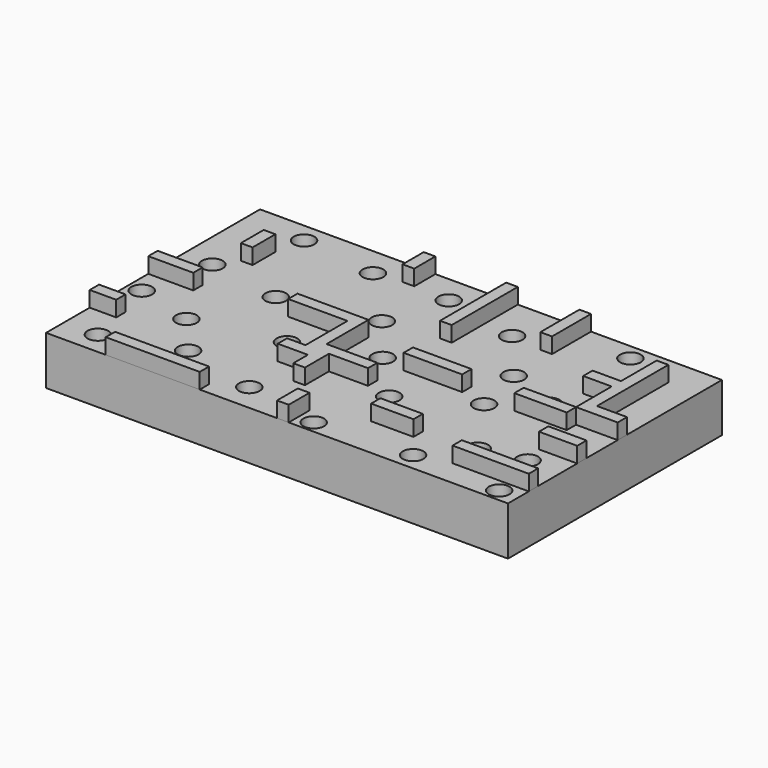
from build123d import *

# Parameters (mm, degrees)
F1_DEPTH = 12.7
F2_R     = 2.7051
F3_DEPTH = 12.701
F4_DEPTH = 12.701
F5_W     = 7.4367895722
F5_H     = 3.048
F6_DEPTH = 4.064
F5_W_2   = 13.6774629354
F5_W_3   = 9.984705162
F5_W_4   = 19.9265140414
F5_W_5   = 11.0705606639
F5_W_6   = 3.048
F5_H_2   = 6.795296824
F5_W_7   = 15.4987806454
F5_H_3   = 7.4474671856
F5_H_4   = 6.8967710249
F5_H_5   = 21.5904228389
F5_H_6   = 12.7339735627
F5_W_8   = 15.297499951
F5_W_9   = 24.5565120131
F5_W_10  = 6.9256495059
F5_W_11  = 11.7564420521


# Not quite as in the source:
# - a feature names something its author has since deleted; it is built from what else it names


with BuildPart() as f1:
    # F0 (on Top) → F1 (new body)
    with BuildSketch(Plane.XY):
        Polygon((0, 0), (-60.325, 0), (-60.325, -69.85), (60.325, -69.85), (60.325, 0), align=None)
    extrude(amount=F1_DEPTH)

    # F2 (on face) → F3 (cut, through all)
    with BuildSketch(Plane.XY.offset(12.7)):
        with Locations((26.0391515287, -25.1232429502)):
            Circle(F2_R)
        with Locations((39.3320303045, -30.1866039911)):
            Circle(F2_R)
        with Locations((51.5670966979, -52.4852229461)):
            Circle(F2_R)
        with Locations((40.3696976448, -54.7941951459)):
            Circle(F2_R)
        with Locations((29.1407505167, -38.6848830029)):
            Circle(F2_R)
        with Locations((39.813039536, -4.2391167363)):
            Circle(F2_R)
        with Locations((14.7792350719, -11.5783627619)):
            Circle(F2_R)
        with Locations((-5.1395187476, -7.3578745587)):
            Circle(F2_R)
        with Locations((-10.0313894829, -23.0711551039)):
            Circle(F2_R)
        with Locations((0.1915656628, -35.5963533331)):
            Circle(F2_R)
        with Locations((11.9079070905, -48.1234616893)):
            Circle(F2_R)
        with Locations((-19.3813890983, -42.3874461546)):
            Circle(F2_R)
        with Locations((-24.7069996912, -7.6543525113)):
            Circle(F2_R)
        with Locations((-33.624197891, -28.248605245)):
            Circle(F2_R)
        with Locations((-32.7827430181, -57.898504717)):
            Circle(F2_R)
        with Locations((-12.9604163302, -62.6995104729)):
            Circle(F2_R)
        with Locations((7.0160373541, -66.6532692993)):
            Circle(F2_R)
        with Locations((31.8740387344, -65.2726447941)):
            Circle(F2_R)
        with Locations((55.3417858057, -66.5050328202)):
            Circle(F2_R)
        with Locations((-41.7826166632, -47.2058818733)):
            Circle(F2_R)
        with Locations((-56.7193522528, -43.1217187759)):
            Circle(F2_R)
        with Locations((-52.6753959628, -25.1232429502)):
            Circle(F2_R)
        with Locations((-44.7191960654, -5.1342979052)):
            Circle(F2_R)
        with Locations((-51.5628442894, -63.8967803387)):
            Circle(F2_R)
    extrude(amount=-F3_DEPTH, mode=Mode.SUBTRACT)

    # F2 (on face) → F4 (cut, through all)
    with BuildSketch(Plane.XY.offset(12.7)):
        with Locations((45.4391605129, -16.2334538194)):
            Circle(F2_R)
    extrude(amount=-F4_DEPTH, mode=Mode.SUBTRACT)


with BuildPart() as f6:
    # F5 (on face) → F6 (new body)
    with BuildSketch(Plane.XY.offset(12.7)):
        Polygon((52.4944375079, -7.7022910118), (49.4464375079, -7.7022910118), (49.4464375079, -19.3477486451), (49.4464375079, -22.3957486451), (49.4464375079, -30.9932062783), (52.4944375079, -30.9932062783), align=None)
        with Locations((45.7280427217, -20.8717486451)):
            Rectangle(F5_W, F5_H)
        Polygon((60.325, -30.9932062783), (52.4944375079, -30.9932062783), (49.4464375079, -30.9932062783), (49.4464375079, -34.0412062783), (60.325, -34.0412062783), align=None)
    extrude(amount=F6_DEPTH)


with BuildPart() as f6b:
    # F5 (on face) → F6, piece 2 (new body)
    with BuildSketch(Plane.XY.offset(12.7)):
        with Locations((42.6077060401, -35.5652062783)):
            Rectangle(F5_W_2, F5_H)
    extrude(amount=F6_DEPTH)


with BuildPart() as f6c:
    # F5 (on face) → F6, piece 3 (new body)
    with BuildSketch(Plane.XY.offset(12.7)):
        with Locations((55.332647419, -45.7249781678)):
            Rectangle(F5_W_3, F5_H)
    extrude(amount=F6_DEPTH)


with BuildPart() as f6d:
    # F5 (on face) → F6, piece 4 (new body)
    with BuildSketch(Plane.XY.offset(12.7)):
        with Locations((50.3617429793, -61.530703176)):
            Rectangle(F5_W_4, F5_H)
    extrude(amount=F6_DEPTH)


with BuildPart() as f6e:
    # F5 (on face) → F6, piece 5 (new body)
    with BuildSketch(Plane.XY.offset(12.7)):
        with Locations((21.3772505522, -57.4178932796)):
            Rectangle(F5_W_5, F5_H)
    extrude(amount=F6_DEPTH)


with BuildPart() as f6f:
    # F5 (on face) → F6, piece 6 (new body)
    with BuildSketch(Plane.XY.offset(12.7)):
        with Locations((1.524, -66.452351588)):
            Rectangle(F5_W_6, F5_H_2)
    extrude(amount=F6_DEPTH)


with BuildPart() as f6g:
    # F5 (on face) → F6, piece 7 (new body)
    with BuildSketch(Plane.XY.offset(12.7)):
        Polygon((-4.6313766771, -47.1245971699), (-7.6793766771, -47.1245971699), (-7.6793766771, -50.1725971699), (-7.6793766771, -54.9458710858), (-4.6313766771, -54.9458710858), align=None)
        Polygon((-7.6793766771, -47.1245971699), (-10.7273766771, -47.1245971699), (-15.5581627041, -47.1245971699), (-15.5581627041, -50.1725971699), (-7.6793766771, -50.1725971699), align=None)
        Polygon((-7.6793766771, -30.3893553474), (-10.7273766771, -30.3893553474), (-10.7273766771, -33.4373553474), (-10.7273766771, -47.1245971699), (-7.6793766771, -47.1245971699), (-7.6793766771, -44.0765971699), align=None)
        Polygon((5.5765425786, -44.0765971699), (-7.6793766771, -44.0765971699), (-7.6793766771, -47.1245971699), (-4.6313766771, -47.1245971699), (5.5765425786, -47.1245971699), align=None)
        with Locations((-18.4767669998, -31.9133553474)):
            Rectangle(F5_W_7, F5_H)
    extrude(amount=F6_DEPTH)


with BuildPart() as f6h:
    # F5 (on face) → F6, piece 8 (new body)
    with BuildSketch(Plane.XY.offset(12.7)):
        with Locations((-47.6484051535, -16.4577062242)):
            Rectangle(F5_W_6, F5_H_3)
    extrude(amount=F6_DEPTH)


with BuildPart() as f6i:
    # F5 (on face) → F6, piece 9 (new body)
    with BuildSketch(Plane.XY.offset(12.7)):
        with Locations((-16.0469947944, -3.4483855125)):
            Rectangle(F5_W_6, F5_H_4)
    extrude(amount=F6_DEPTH)


with BuildPart() as f6j:
    # F5 (on face) → F6, piece 10 (new body)
    with BuildSketch(Plane.XY.offset(12.7)):
        with Locations((5.4902756026, -10.7952114195)):
            Rectangle(F5_W_6, F5_H_5)
    extrude(amount=F6_DEPTH)


with BuildPart() as f6k:
    # F5 (on face) → F6, piece 11 (new body)
    with BuildSketch(Plane.XY.offset(12.7)):
        with Locations((24.612151589, -6.3669867814)):
            Rectangle(F5_W_6, F5_H_6)
    extrude(amount=F6_DEPTH)


with BuildPart() as f6l:
    # F5 (on face) → F6, piece 12 (new body)
    with BuildSketch(Plane.XY.offset(12.7)):
        with Locations((14.6630255781, -35.7664874384)):
            Rectangle(F5_W_8, F5_H)
    extrude(amount=F6_DEPTH)


with BuildPart() as f6m:
    # F5 (on face) → F6, piece 13 (new body)
    with BuildSketch(Plane.XY.offset(12.7)):
        with Locations((-32.4659263715, -68.326)):
            Rectangle(F5_W_9, F5_H)
    extrude(amount=F6_DEPTH)


with BuildPart() as f6n:
    # F5 (on face) → F6, piece 14 (new body)
    with BuildSketch(Plane.XY.offset(12.7)):
        with Locations((-56.8621752471, -54.0832294712)):
            Rectangle(F5_W_10, F5_H)
    extrude(amount=F6_DEPTH)


with BuildPart() as f6o:
    # F5 (on face) → F6, piece 15 (new body)
    with BuildSketch(Plane.XY.offset(12.7)):
        with Locations((-54.4467789739, -34.9613553474)):
            Rectangle(F5_W_11, F5_H)
    extrude(amount=F6_DEPTH)


solid = Compound([f1.part, f6.part, f6b.part, f6c.part, f6d.part, f6e.part, f6f.part, f6g.part, f6h.part, f6i.part, f6j.part, f6k.part, f6l.part, f6m.part, f6n.part, f6o.part])
